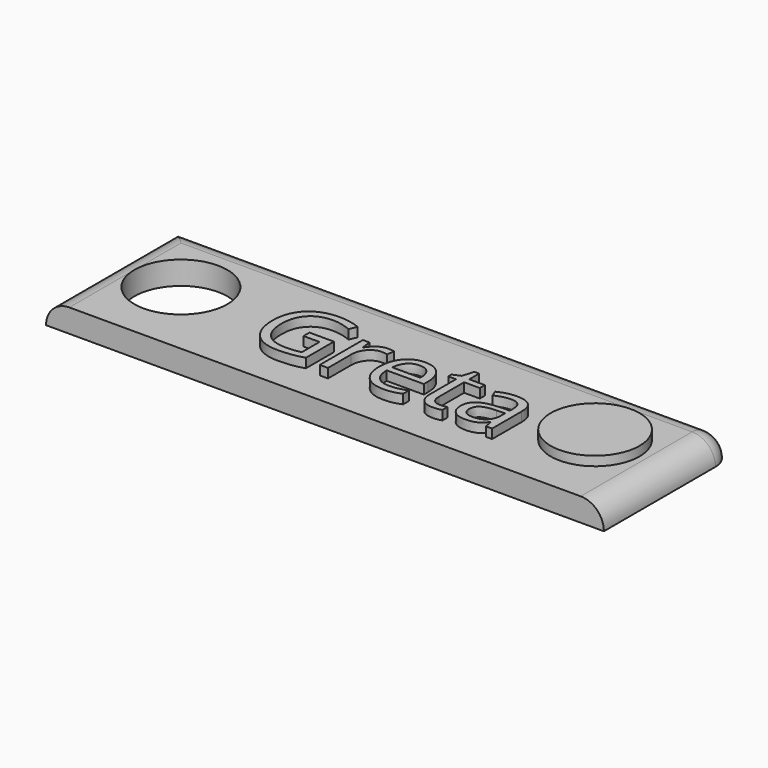
from build123d import *

# Parameters (mm, degrees)
F0_W         = 120
F0_H         = 35
F0_R         = 10
F1_DEPTH     = 5
F2_R         = 4.99999
F3_R         = 4.99999
F4_TEXT_SIZE = 21.6559603966
F5_DEPTH     = 2
F6_R         = 9.5565861829
F7_DEPTH     = 2


# Not quite as in the source:
# - a fillet or chamfer is up to 0.001 mm smaller than in the source, because OpenCascade refuses the exact size
# - Text() gives the source's letters only with a copy of the font that has no kerning and outlines rounded to 1/6400 em; it was checked with that copy


with BuildPart() as f1:
    # F0 (on Top) → F1 (new body)
    with BuildSketch(Plane.XY):
        Rectangle(F0_W, F0_H)
        with Locations((-45, 0)):
            Circle(F0_R, mode=Mode.SUBTRACT)
    extrude(amount=F1_DEPTH)

    # F2 (radius 5 in the source; OpenCascade refuses exactly that, so slightly less here)
    f2_edges = [f1.edges().sort_by_distance(p)[0] for p in [
        (-60, 0, 5),
        (0, 17.5, 5),
    ]]
    fillet(f2_edges, radius=F2_R)

    # F3 (radius 5 in the source; OpenCascade refuses exactly that, so slightly less here)
    f3_edges = [f1.edges().sort_by_distance(p)[0] for p in [
        (60, -2.499995, 5),
    ]]
    fillet(f3_edges, radius=F3_R)

    # F4 (on face) → F5 (join)
    with BuildSketch(Plane.XY.offset(5)):
        with Locations((-24.3056323379, -10.547732003)):
            Text('Greta', F4_TEXT_SIZE, font='Open Sans', text_align=(TextAlign.LEFT, TextAlign.BOTTOM))
    extrude(amount=F5_DEPTH)

    # F6 (on face) → F7 (join)
    with BuildSketch(Plane.XY.offset(5)):
        with Locations((44.1118441522, 0)):
            Circle(F6_R)
    extrude(amount=F7_DEPTH)


solid = f1.part
